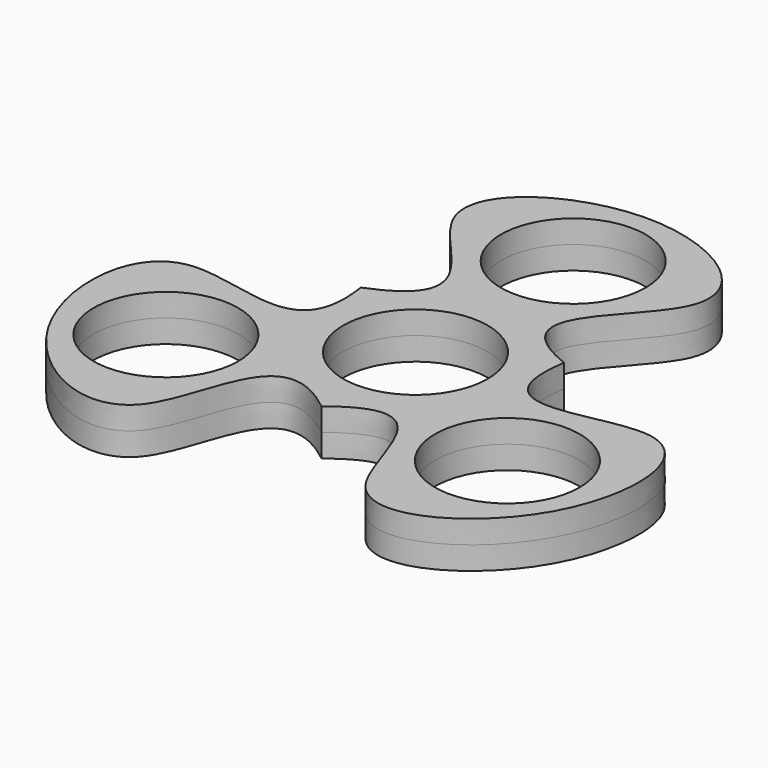
from build123d import *

# Parameters (mm, degrees)
F0_R     = 11
F1_DEPTH = 3.5


# Not quite as in the source:
# - ends of sketch curves that miss each other by under 0.0002 mm in the source are joined


with BuildPart() as f1:
    # F0 (on Top) → F1 (new body, symmetric)
    with BuildSketch(Plane.XY):
        with BuildLine():
            add(Edge.make_bspline(
                [(0.0001862709, -17.854371812), (-12.9900730105, -7.5006266371), (-11.2804815695, -42.4870572563), (-43.9678605577, -25.3855549258), (-42.4345050326, 11.4733326926), (-12.9900780334, -7.5005238465), (-15.4616634595, 8.9264466646)],
                knots=[7.345e-07, 7.345e-07, 7.345e-07, 7.345e-07, 0.2451705527, 0.5, 0.7548294473, 1, 1, 1, 1], degree=3))
            add(Edge.make_bspline(
                [(15.4619664829, 8.9269705111), (12.9908834331, -7.5002900471), (42.4361006075, 11.4722752907), (43.9651206921, -25.3804304153), (11.2943720802, -42.5045779891), (12.96372192, -7.4636177935), (0.0001862709, -17.854371812)],
                knots=[0, 0, 0, 0, 0.2451727415, 0.5000010107, 0.7548292798, 0.9999986639, 0.9999986639, 0.9999986639, 0.9999986639], degree=3))
            add(Edge.make_bspline(
                [(-15.4616634595, 8.9264466646), (0, 15), (-31.1540001349, 31.0125066494), (-3.16279e-05, 50.7701004871), (31.1539286772, 31.0126855588), (0.0003516695, 15.0001807525), (15.4619664829, 8.9269705111)],
                knots=[0, 0, 0, 0, 0.2451726624, 0.5000009582, 0.7548292541, 0.999997178, 0.999997178, 0.999997178, 0.999997178], degree=3))
        make_face()
        with Locations((-25.9807621135, -15.0005800942)):
            Circle(F0_R, mode=Mode.SUBTRACT)
        Circle(F0_R, mode=Mode.SUBTRACT)
        with Locations((25.9812644899, -15.0002900471)):
            Circle(F0_R, mode=Mode.SUBTRACT)
        with Locations((0, 30)):
            Circle(F0_R, mode=Mode.SUBTRACT)
    extrude(amount=F1_DEPTH, both=True)


solid = f1.part
